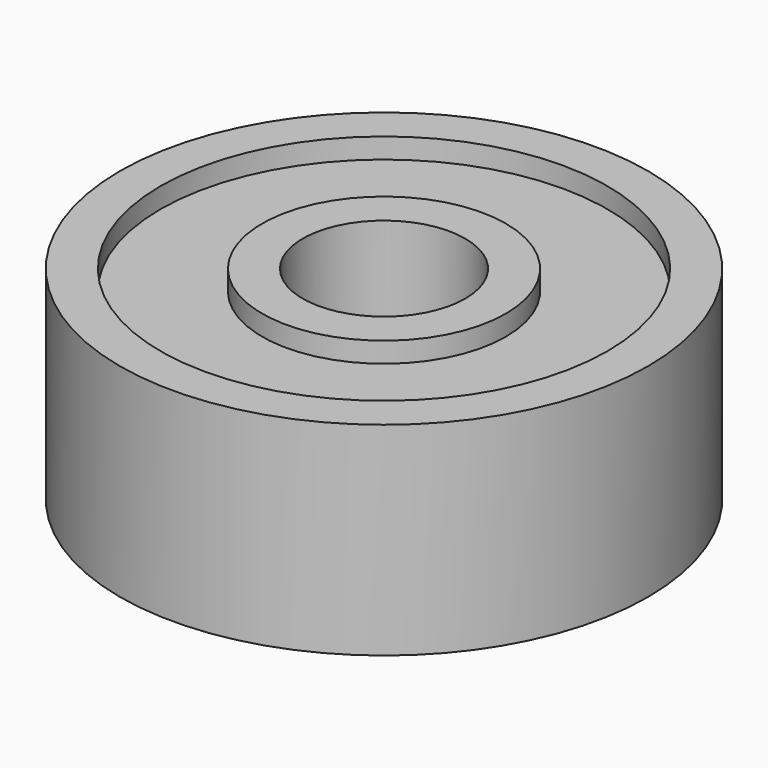
from build123d import *

# Parameters (mm, degrees)
F0_R     = 6.5
F0_R_2   = 5.5
F1_DEPTH = 2.5
F0_R_3   = 3
F0_R_4   = 2
F2_DEPTH = 2


with BuildPart() as f1:
    # F0 (on Top) → F1 (new body, symmetric)
    with BuildSketch(Plane.XY):
        Circle(F0_R)
        Circle(F0_R_2, mode=Mode.SUBTRACT)
    extrude(amount=F1_DEPTH, both=True)



with BuildPart() as f1b:
    # F0 (on Top) → F1, piece 2 (new body, symmetric)
    with BuildSketch(Plane.XY):
        Circle(F0_R_3)
        Circle(F0_R_4, mode=Mode.SUBTRACT)
    extrude(amount=F1_DEPTH, both=True)


with BuildPart() as f1_1:
    add(f1.part)

    add(f1b.part)  # F2 merges F1b
    # F0 (on Top) → F2 (join, symmetric)
    with BuildSketch(Plane.XY):
        Circle(F0_R_2)
        Circle(F0_R_3, mode=Mode.SUBTRACT)
    extrude(amount=F2_DEPTH, both=True)


solid = f1_1.part
